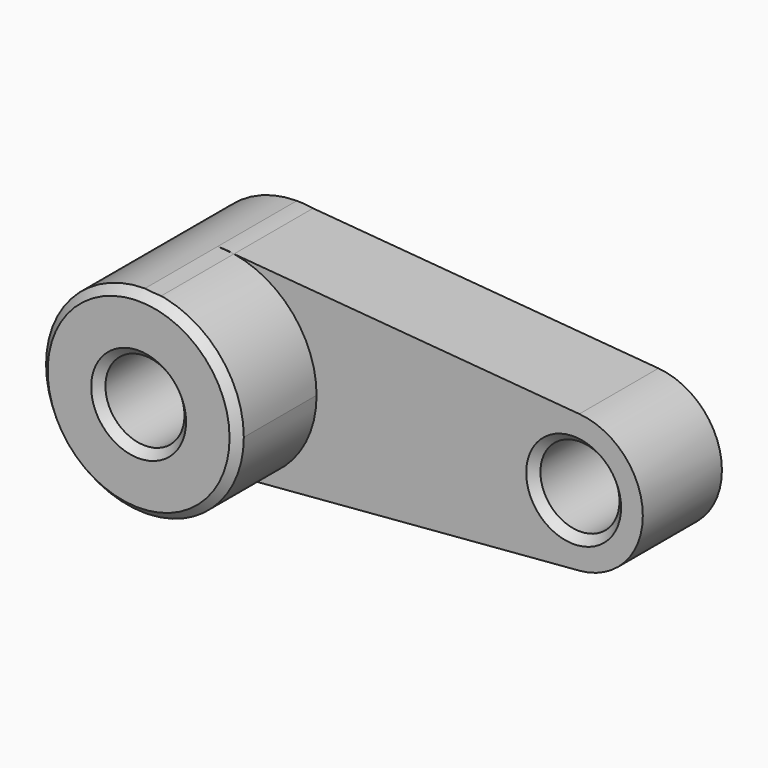
from build123d import *

# Parameters (mm, degrees)
F0_R        = 10
F1_DEPTH    = 25
F2_DEPTH    = 50
F3_T4_ANGLE = 203.6133668192
F3_T6_ANGLE = 179.9906971182


# Not quite as in the source:
# - a fillet or chamfer that OpenCascade refuses, or shapes differently, is made with other operations: its cross-section is extruded or revolved along the edge and cut away or added


with BuildPart() as f1:
    # F0 (on Front) → F1 (new body)
    with BuildSketch(Plane.XZ):
        with BuildLine():
            Line((4.1054428346, 24.6606029758), (0, 25))
            ThreePointArc((0, 25), (-25, 0), (0, -25))
            Line((0, -25), (4.1054428346, -24.6606029758))
            ThreePointArc((4.1054428346, -24.6606029758), (19.0740146648, -16.1611251022), (25, 0))
            ThreePointArc((25, 0), (19.0740146648, 16.1611251022), (4.1054428346, 24.6606029758))
        make_face()
        Circle(F0_R, mode=Mode.SUBTRACT)
        with BuildLine():
            ThreePointArc((4.1054428346, 24.6606029758), (2.0597239626, 24.9150062653), (0, 25))
            Line((0, 25), (4.1054428346, 24.6606029758))
        make_face()
        with BuildLine():
            Line((4.1054428346, -24.6606029758), (0, -25))
            ThreePointArc((0, -25), (2.0597239626, -24.9150062653), (4.1054428346, -24.6606029758))
        make_face()
        with BuildLine():
            Line((91.4418067738, 17.4405043857), (4.1054428346, 24.6606029758))
            ThreePointArc((4.1054428346, 24.6606029758), (19.0740146648, 16.1611251022), (25, 0))
            ThreePointArc((25, 0), (19.0740146648, -16.1611251022), (4.1054428346, -24.6606029758))
            Line((4.1054428346, -24.6606029758), (91.4418067738, -17.4405043857))
            ThreePointArc((91.4418067738, -17.4405043857), (72.5, 0), (91.4418067738, 17.4405043857))
        make_face()
        with BuildLine():
            ThreePointArc((107.5, 0), (102.8740362463, 11.8536572723), (91.4418067738, 17.4405043857))
            ThreePointArc((91.4418067738, 17.4405043857), (72.5, 0), (91.4418067738, -17.4405043857))
            ThreePointArc((91.4418067738, -17.4405043857), (102.8740362463, -11.8536572723), (107.5, 0))
        make_face()
        with Locations((90, 0)):
            Circle(F0_R, mode=Mode.SUBTRACT)
    extrude(amount=F1_DEPTH)

    # F0 (on Front) → F2 (join)
    with BuildSketch(Plane.XZ):
        with BuildLine():
            Line((4.1054428346, 24.6606029758), (0, 25))
            ThreePointArc((0, 25), (-25, 0), (0, -25))
            Line((0, -25), (4.1054428346, -24.6606029758))
            ThreePointArc((4.1054428346, -24.6606029758), (19.0740146648, -16.1611251022), (25, 0))
            ThreePointArc((25, 0), (19.0740146648, 16.1611251022), (4.1054428346, 24.6606029758))
        make_face()
        Circle(F0_R, mode=Mode.SUBTRACT)
    extrude(amount=F2_DEPTH)

    # F3: chamfer of 2 on 5 edges, made by hand

    # F3_s1 → F3_t2 (revolve, cut)
    with BuildSketch(Plane.XY):
        Polygon((12, -50), (10, -48), (10, -50), align=None)
    revolve(axis=Axis((0, -50, 0), (0, -1, 0)), mode=Mode.SUBTRACT)

    # F3_s3 → F3_t4 (revolve, cut)
    with BuildSketch(Plane(origin=(0, 0, 0), x_dir=(0, 1, 0), z_dir=(0.9788435281, 0, -0.2046102329))):
        Polygon((-48, 25), (-50, 23), (-50, 25), align=None)
    revolve(axis=Axis((0, -50, 0), (0, -1, 0)), revolution_arc=F3_T4_ANGLE, mode=Mode.SUBTRACT)

    # F3_s5 → F3_t6 (revolve, cut)
    with BuildSketch(Plane(origin=(0, 0, 0), x_dir=(0, 1, 0), z_dir=(-0.9999999967, 0, 8.1183e-05))):
        Polygon((-48, -25), (-50, -23), (-50, -25), align=None)
    revolve(axis=Axis((0, -50, 0), (0, 1, 0)), revolution_arc=F3_T6_ANGLE, mode=Mode.SUBTRACT)

    # F3_s7 → F3_t8 (revolve, cut)
    with BuildSketch(Plane.XY):
        Polygon((100, -2), (102, 0), (100, 0), align=None)
    revolve(axis=Axis((90, 0, 0), (0, -1, 0)), mode=Mode.SUBTRACT)

    # F3_s9 → F3_t10 (revolve, cut)
    with BuildSketch(Plane.XY):
        Polygon((102, -25), (100, -23), (100, -25), align=None)
    revolve(axis=Axis((90, -25, 0), (0, -1, 0)), mode=Mode.SUBTRACT)


solid = f1.part
